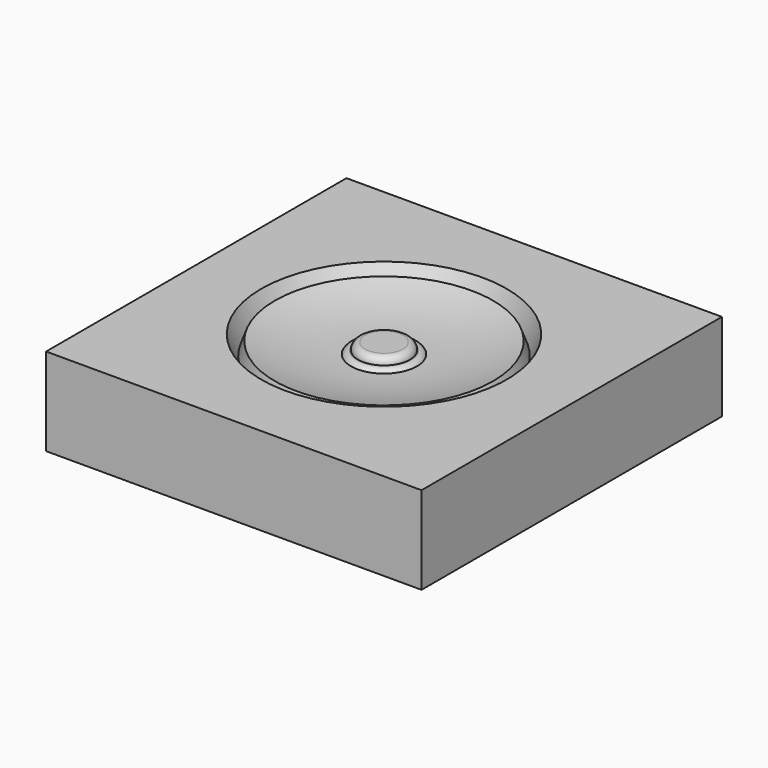
from build123d import *

# Parameters (mm, degrees)
F0_W     = 135.89
F0_H     = 135.89
F1_DEPTH = 31.75


# Not quite as in the source:
# - a fillet or chamfer that OpenCascade refuses, or shapes differently, is made with other operations: its cross-section is extruded or revolved along the edge and cut away or added


with BuildPart() as f1:
    # F0 (on Top) → F1 (new body)
    with BuildSketch(Plane.XY):
        Rectangle(F0_W, F0_H)
    extrude(amount=F1_DEPTH)

    # F2 (on Front) → F3 (revolve, cut)
    with BuildSketch(Plane.XZ):
        with BuildLine():
            Line((0, 29.21), (0, 31.75))
            Line((0, 31.75), (-44.45, 31.75))
            Line((-44.45, 31.75), (-41.2296488455, 24.8439346628))
            Line((-41.2296488455, 24.8439346628), (-39.4921865174, 29.6175731764))
            ThreePointArc((-39.4921865174, 29.6175731764), (-25.8683470518, 26.5354678002), (-11.9464546442, 25.4))
            Line((-11.9464546442, 25.4), (-11.9464546442, 26.67))
            Line((-11.9464546442, 26.67), (-9.398, 26.67))
            Line((-9.398, 26.67), (-9.398, 29.21))
            Line((-9.398, 29.21), (0, 29.21))
        make_face()
    revolve(axis=Axis((0, 0, 21.6028230067), (0, 0, -1)), mode=Mode.SUBTRACT)

    # F4: fillet of radius 2.54 on 2 edges, made by hand

    # F4_s1 → F4_t2 (revolve, cut)
    with BuildSketch(Plane.XZ):
        with BuildLine():
            ThreePointArc((-9.398, 26.67), (-8.6540512242, 28.4660512242), (-6.858, 29.21))
            Line((-6.858, 29.21), (-9.398, 29.21))
            Line((-9.398, 29.21), (-9.398, 26.67))
        make_face()
    revolve(axis=Axis((0, 0, 29.21), (0, 0, -1)), mode=Mode.SUBTRACT)

    # F4_s3 → F4_t4 (revolve, cut)
    with BuildSketch(Plane.XZ):
        with BuildLine():
            ThreePointArc((-11.9464546442, 25.4), (-11.0167501186, 26.3297045256), (-9.7467501186, 26.67))
            Line((-9.7467501186, 26.67), (-11.9464546442, 26.67))
            Line((-11.9464546442, 26.67), (-11.9464546442, 25.4))
        make_face()
    revolve(axis=Axis((0, 0, 26.67), (0, 0, -1)), mode=Mode.SUBTRACT)


solid = f1.part
